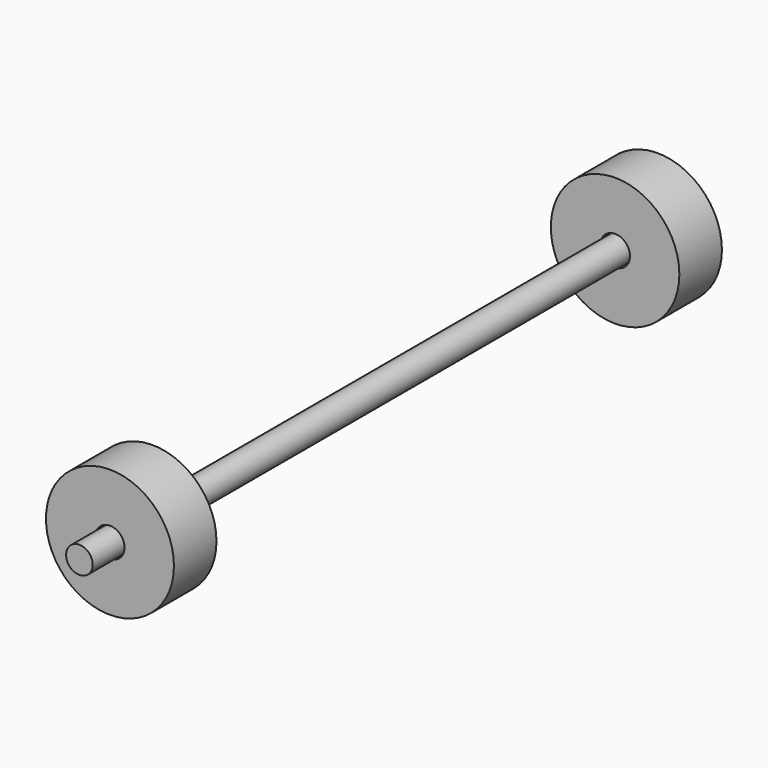
from build123d import *

# Parameters (mm, degrees)
F2_R      = 8.4099565343
F4_DEPTH  = 6.99204
F3_R      = 1.919597314
F5_DEPTH  = 7.58419
F6_R      = 1.75
F7_DEPTH  = 50.00907
F8_R      = 8.4466451415
F10_DEPTH = 6.992
F9_R      = 1.9516228475
F11_DEPTH = 10.0613
F12_DEPTH = 50.009


# Not quite as in the source:
# - a feature names something its author has since deleted; it is built from what else it names


with BuildPart() as f4:
    # F2 (on offset) → F4 (new body)
    with BuildSketch(Plane.XZ.offset(38)):
        Circle(F2_R)
    extrude(amount=F4_DEPTH)

    # F3 (on offset) → F5 (cut)
    with BuildSketch(Plane.XZ.offset(38)):
        Circle(F3_R)
    extrude(amount=F5_DEPTH, mode=Mode.SUBTRACT)


with BuildPart() as f7:
    # F6 (on Front) → F7 (new body)
    with BuildSketch(Plane.XZ):
        Circle(F6_R)
    extrude(amount=F7_DEPTH)

    # F6 (on Front) → F12 (join)
    with BuildSketch(Plane.XZ):
        Circle(F6_R)
    extrude(amount=-F12_DEPTH)


with BuildPart() as f10:
    # F8 (on offset) → F10 (new body)
    with BuildSketch(Plane.XZ.offset(-38)):
        Circle(F8_R)
    extrude(amount=-F10_DEPTH)

    # F9 (on offset) → F11 (cut)
    with BuildSketch(Plane.XZ.offset(-38)):
        Circle(F9_R)
    extrude(amount=-F11_DEPTH, mode=Mode.SUBTRACT)


solid = Compound([f4.part, f7.part, f10.part])
